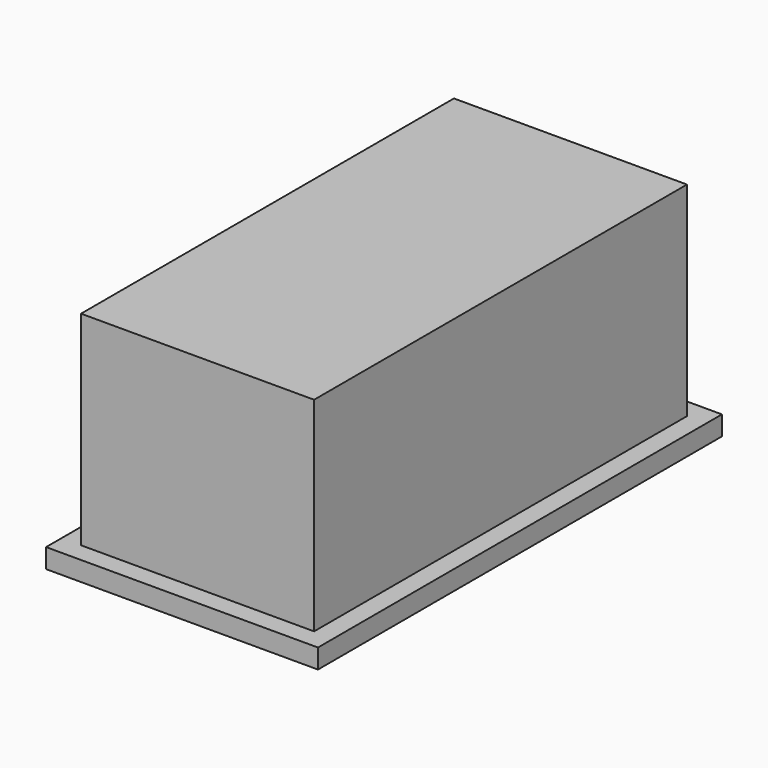
from build123d import *

# Parameters (mm, degrees)
F0_W         = 1219.2
F0_H         = 1066.8
F1_DEPTH     = 2438.4
F3_DEPTH     = 2540
F4_DEPTH     = 101.6
F5_TEXT_SIZE = 309.8132295741
F6_DEPTH     = 25.4


# Not quite as in the source:
# - Text() gives the source's letters only with a copy of the font that has no kerning and outlines rounded to 1/6400 em; it was checked with that copy


with BuildPart() as f1:
    # F0 (on Front) → F1 (new body)
    with BuildSketch(Plane.XZ):
        with Locations((542.0699931952, 515.1206709862)):
            Rectangle(F0_W, F0_H)
    extrude(amount=F1_DEPTH)

    # F5 (on face) → F6 (join)
    with BuildSketch(Plane(origin=(-67.5300068048, 0, 0), x_dir=(0, -1, 0), z_dir=(-1, 0, 0))):
        with Locations((88.6816978455, 68.9205005765)):
            Text('AHU-AQE-1', F5_TEXT_SIZE, font='Open Sans', text_align=(TextAlign.LEFT, TextAlign.BOTTOM))
    extrude(amount=F6_DEPTH)


with BuildPart() as f3:
    # F2 (on face) → F3 (new body)
    with BuildSketch(Plane.XZ.offset(2438.4)):
        Polygon((-67.5300068048, -18.2793290138), (-169.1300068048, -18.2793290138), (-169.1300068048, -119.8793290138), (1253.2699931952, -119.8793290138), (1253.2699931952, -18.2793290138), (1151.6699931952, -18.2793290138), align=None)
    extrude(amount=-F3_DEPTH)

    # F4 (add): a face of the model
    f4_faces = [f3.faces().sort_by_distance(p)[0] for p in [
        (542.0699931952, -2438.4, -69.0793290138),
    ]]
    extrude(f4_faces, amount=F4_DEPTH)


solid = Compound([f1.part, f3.part])
